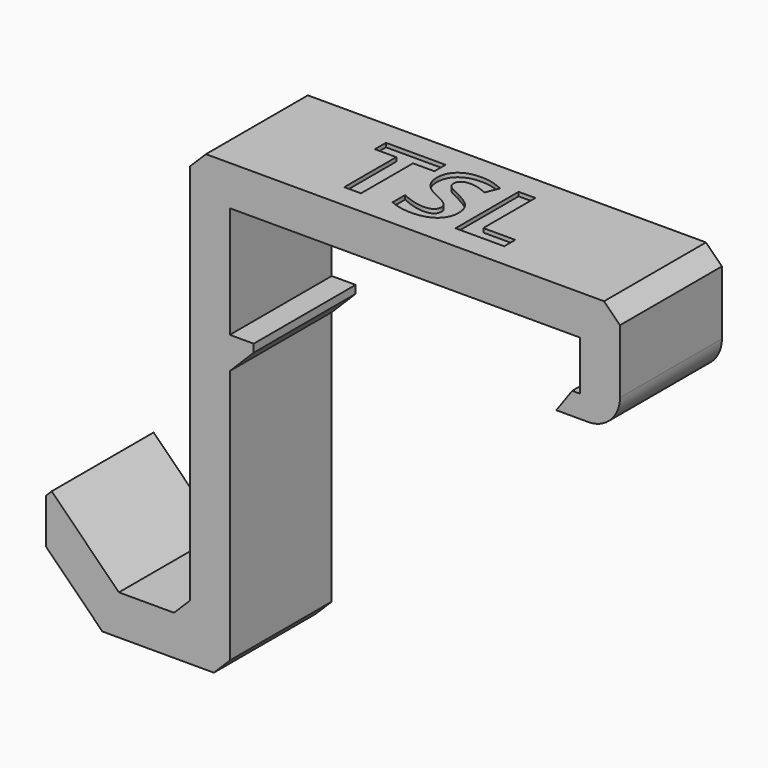
from build123d import *

# Parameters (mm, degrees)
F1_DEPTH     = 8
F2_T1_DEPTH  = 18.2867319519
F2_T6_DEPTH  = 18.2867319519
F3_R         = 2
F4_SIZE      = 1
F5_TEXT_SIZE = 6.9444444444
F6_DEPTH     = 0.25


# Not quite as in the source:
# - a fillet or chamfer that OpenCascade refuses, or shapes differently, is made with other operations: its cross-section is extruded or revolved along the edge and cut away or added
# - Text() gives the source's letters only with a copy of the font that has no kerning and outlines rounded to 1/6400 em; it was checked with that copy


with BuildPart() as f1:
    # F0 (on Front) → F1 (new body)
    with BuildSketch(Plane.XZ):
        Polygon((-0.5, 18.5), (-0.5, 25.5), (21.5, 25.5), (21.5, 22.4), (21, 22.4), (20, 21), (24, 21), (24, 22.4), (24, 28), (21.5, 28), (-0.5, 28), (-3, 28), (-3, 25.5), (-3, 2), (-7.4644660941, 2), (-11.6819805153, 6.2175144213), (-13.4497474683, 4.4497474683), (-8.5, -0.5), (-0.5, -0.5), (-0.5, 16), (1, 16), (1, 18.5), align=None)
    extrude(amount=F1_DEPTH)

    # F2: chamfer of 2 on 2 edges, made by hand

    # F2_s2 → F2_t1 (cut)
    with BuildSketch(Plane.XZ.offset(-5.1433659759)):
        Polygon((-12.0355339059, 5.8639610307), (-12.0355339059, 3.0355339059), (-13.4497474683, 4.4497474683), align=None)
    extrude(amount=F2_T1_DEPTH, mode=Mode.SUBTRACT)


with BuildPart() as f2_tool4:
    # F2_s5 → F2_t6 (new body)
    with BuildSketch(Plane.XZ.offset(-5.1433659759)):
        Polygon((1, 18), (-1, 16), (1, 16), align=None)
    extrude(amount=F2_T6_DEPTH)

    split(bisect_by=Plane.YZ.offset(-0.5), keep=Keep.TOP)


with BuildPart() as f1_1:
    add(f1.part)

    # F2_t3: cut F2_tool4
    add(f2_tool4.part, mode=Mode.SUBTRACT)

    # F3
    f3_edges = [f1_1.edges().sort_by_distance(p)[0] for p in [
        (24, -4, 21),
    ]]
    fillet(f3_edges, radius=F3_R)

    # F4
    f4_edges = [f1_1.edges().sort_by_distance(p)[0] for p in [
        (-0.5, -4, -0.5),
        (-3, -4, 2),
        (24, -4, 28),
        (-3, -4, 28),
    ]]
    chamfer(f4_edges, length=F4_SIZE)

    # F5 (on face) → F6 (cut)
    with BuildSketch(Plane.XY.offset(28)):
        with Locations((4, -6.5)):
            Text('TSL', F5_TEXT_SIZE, font='Open Sans', font_style=FontStyle.BOLD, text_align=(TextAlign.LEFT, TextAlign.BOTTOM))
    extrude(amount=-F6_DEPTH, mode=Mode.SUBTRACT)


solid = f1_1.part
